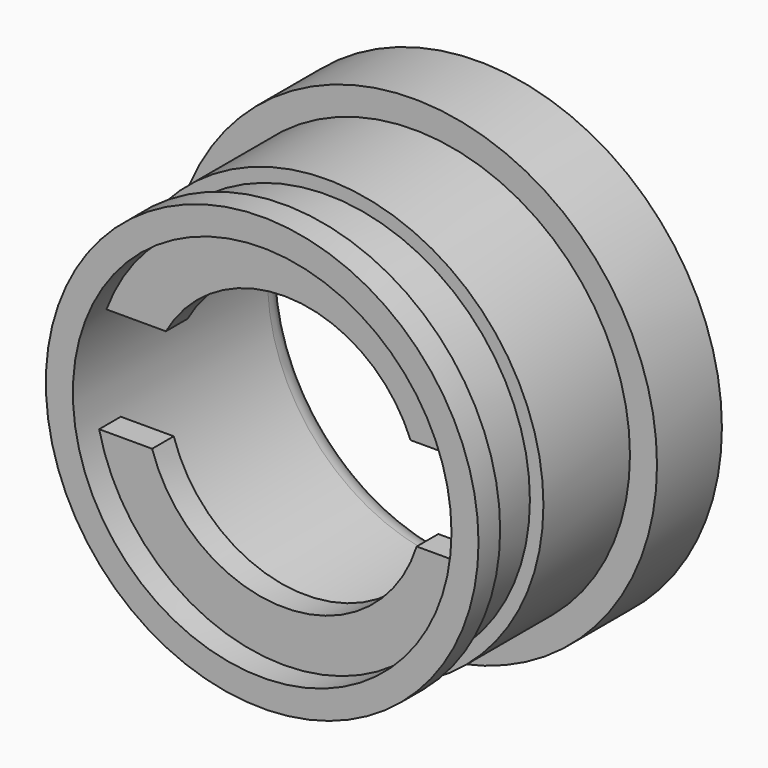
from build123d import *

# Parameters (mm, degrees)
F0_R      = 40
F0_R_2    = 35
F1_DEPTH  = 50
F2_R      = 45
F2_R_2    = 35
F3_DEPTH  = 15
F4_R      = 5
F6_R      = 40
F6_R_2    = 37.5
F7_DEPTH  = 10
F9_DEPTH  = 5
F11_DEPTH = 5


with BuildPart() as f1:
    # F0 (on Front) → F1 (new body)
    with BuildSketch(Plane.XZ):
        Circle(F0_R)
        Circle(F0_R_2, mode=Mode.SUBTRACT)
    extrude(amount=F1_DEPTH)

    # F2 (on Front) → F3 (join)
    with BuildSketch(Plane.XZ):
        Circle(F2_R)
        Circle(F2_R_2, mode=Mode.SUBTRACT)
    extrude(amount=F3_DEPTH)

    # F4
    f4_edges = [f1.edges().sort_by_distance(p)[0] for p in [
        (-35, 0, 0),
    ]]
    fillet(f4_edges, radius=F4_R)

    # F6 (on offset) → F7 (cut)
    with BuildSketch(Plane.XZ.offset(45)):
        Circle(F6_R)
        Circle(F6_R_2, mode=Mode.SUBTRACT)
    extrude(amount=-F7_DEPTH, mode=Mode.SUBTRACT)

    # F8 (on offset) → F9 (join)
    with BuildSketch(Plane.XZ.offset(45)):
        with BuildLine():
            Line((23.4356336296, 9.2309236786), (33.7607767689, 9.2309236786))
            ThreePointArc((33.7607767689, 9.2309236786), (1.5790357434, 34.9643625156), (-32.7912801838, 12.2365004764))
            Line((-32.7912801838, 12.2365004764), (-21.8026206791, 12.2365004764))
            ThreePointArc((-21.8026206791, 12.2365004764), (1.7678734782, 25.0531540072), (23.4356336296, 9.2309236786))
        make_face()
    extrude(amount=-F9_DEPTH)

    # F10 (on offset) → F11 (join)
    with BuildSketch(Plane.XZ.offset(45)):
        with BuildLine():
            Line((-24.3510891636, -7.7079934607), (-34.1406918033, -7.7079934607))
            ThreePointArc((-34.1406918033, -7.7079934607), (0, -35), (34.1406918033, -7.7079934607))
            Line((34.1406918033, -7.7079934607), (24.5616502176, -7.7079934607))
            ThreePointArc((24.5616502176, -7.7079934607), (0.105280527, -25.6222077044), (-24.3510891636, -7.7079934607))
        make_face()
    extrude(amount=-F11_DEPTH)


solid = f1.part
